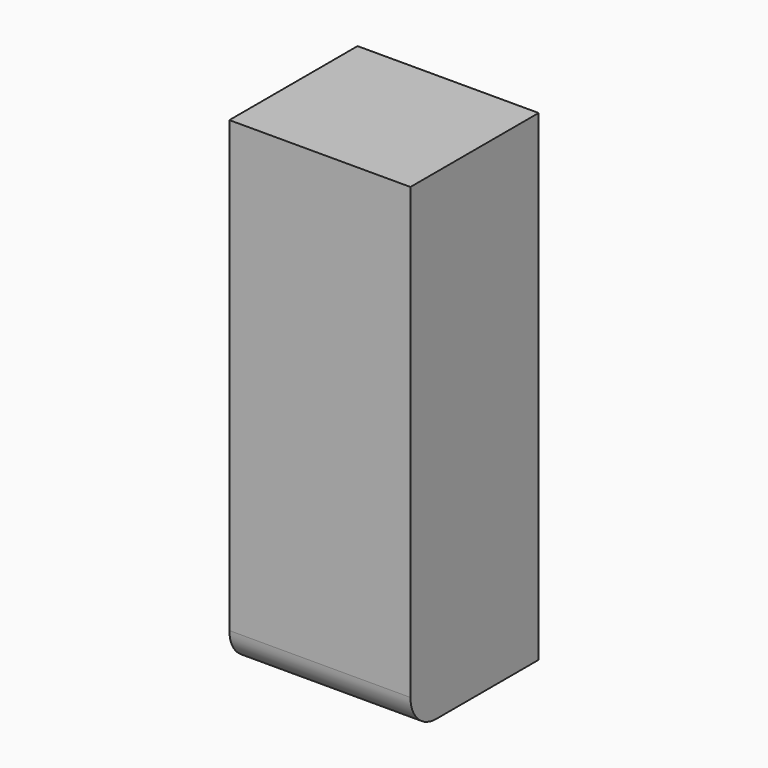
from build123d import *

# Parameters (mm, degrees)
F1_W     = 28.2473526895
F1_H     = 75.105600059
F2_DEPTH = 25
F3_R     = 5


with BuildPart() as f2:
    # F1 (on Front) → F2 (new body)
    with BuildSketch(Plane.XZ):
        with Locations((56.8322334439, 127.3941583931)):
            Rectangle(F1_W, F1_H)
    extrude(amount=F2_DEPTH)

    # F3
    f3_edges = [f2.edges().sort_by_distance(p)[0] for p in [
        (56.832233, -25, 89.841358),
    ]]
    fillet(f3_edges, radius=F3_R)


solid = f2.part
